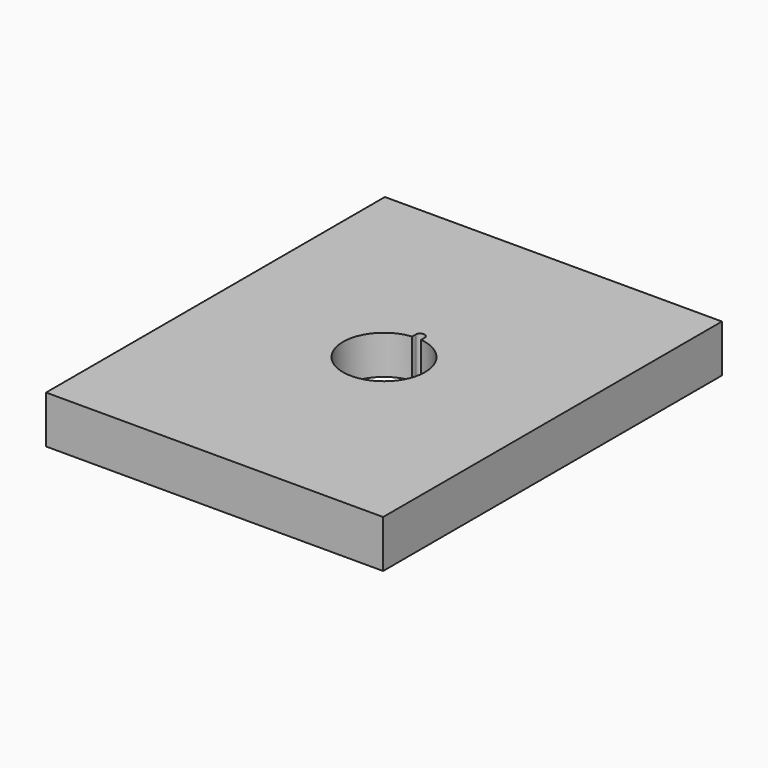
from build123d import *

# Parameters (mm, degrees)
F0_W     = 156
F0_H     = 196
F1_DEPTH = 22
F2_DEPTH = 4
F3_R     = 45
F4_DEPTH = 4


# Not quite as in the source:
# - ends of sketch curves that miss each other by under 0.0002 mm in the source are joined


with BuildPart() as f1:
    # F0 (on Top) → F1 (new body)
    with BuildSketch(Plane.XY):
        with Locations((0.9172109421, 20.8848945383)):
            Rectangle(F0_W, F0_H)
        with BuildLine():
            ThreePointArc((2.9672109421, 39.7739786876), (0.9172109421, 1.8848945383), (-1.1327890579, 39.7739786876))
            Line((-1.1327890579, 39.7739786876), (-1.1327890579, 41.8294366129))
            ThreePointArc((-1.1327890579, 41.8294366129), (0.914481977, 43.8848999875), (2.9672182077, 41.8348945383))
            Line((2.9672182077, 41.8348945383), (2.9672109421, 41.8294366129))
            Line((2.9672109421, 41.8294366129), (2.9672109421, 39.7739786876))
        make_face(mode=Mode.SUBTRACT)
    extrude(amount=F1_DEPTH)

    # F0 (on Top) → F2 (join)
    with BuildSketch(Plane.XY):
        with Locations((0.9172109421, 20.8848945383)):
            Rectangle(F0_W, F0_H)
        with BuildLine():
            ThreePointArc((2.9672109421, 39.7739786876), (0.9172109421, 1.8848945383), (-1.1327890579, 39.7739786876))
            Line((-1.1327890579, 39.7739786876), (-1.1327890579, 41.8294366129))
            ThreePointArc((-1.1327890579, 41.8294366129), (0.914481977, 43.8848999875), (2.9672182077, 41.8348945383))
            Line((2.9672182077, 41.8348945383), (2.9672109421, 41.8294366129))
            Line((2.9672109421, 41.8294366129), (2.9672109421, 39.7739786876))
        make_face(mode=Mode.SUBTRACT)
    extrude(amount=F2_DEPTH)

    # F3 (on face) → F4 (cut)
    with BuildSketch(Plane(origin=(0, 0, 0), x_dir=(1, 0, 0), z_dir=(0, 0, -1))):
        with Locations((0.9172109421, -20.8848945383)):
            Circle(F3_R)
    extrude(amount=-F4_DEPTH, mode=Mode.SUBTRACT)


solid = f1.part
